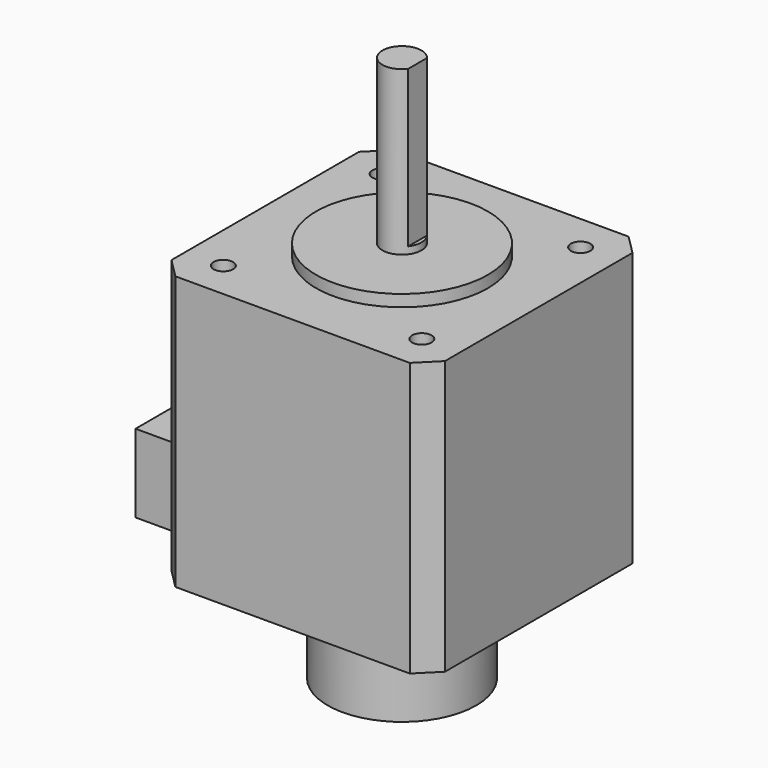
from build123d import *

# Parameters (mm, degrees)
F0_W      = 35
F0_H      = 35
F1_DEPTH  = 35
F2_SIZE   = 2.5
F3_R      = 11
F4_DEPTH  = 1.5
F5_R      = 2.5
F6_DEPTH  = 0.9
F7_W      = 16.5
F7_H      = 10
F8_DEPTH  = 10
F10_DEPTH = 20
F12_D     = 2.5
F12_DEPTH = 4.5
F12_TIP   = 0.7510757738
F20_R     = 9.5
F20_R_2   = 2.5
F21_DEPTH = 12.5
F22_DEPTH = 7.5


with BuildPart() as f1:
    # F0 (on Top) → F1 (new body)
    with BuildSketch(Plane.XY):
        Rectangle(F0_W, F0_H)
    extrude(amount=F1_DEPTH)

    # F2
    f2_edges = [f1.edges().sort_by_distance(p)[0] for p in [
        (17.5, -17.5, 17.5),
        (-17.5, -17.5, 17.5),
        (-17.5, 17.5, 17.5),
        (17.5, 17.5, 17.5),
    ]]
    chamfer(f2_edges, length=F2_SIZE)

    # F3 (on face) → F4 (join)
    with BuildSketch(Plane.XY.offset(35)):
        Circle(F3_R)
    extrude(amount=F4_DEPTH)

    # F5 (on face) → F6 (join)
    with BuildSketch(Plane.XY.offset(36.5)):
        Circle(F5_R)
    extrude(amount=F6_DEPTH)

    # F7 (on face) → F8 (join)
    with BuildSketch(Plane(origin=(-17.5, 0, 0), x_dir=(0, -1, 0), z_dir=(-1, 0, 0))):
        with Locations((0, 5)):
            Rectangle(F7_W, F7_H)
    extrude(amount=F8_DEPTH)

    # F9 (on face) → F10 (join)
    with BuildSketch(Plane.XY.offset(37.4)):
        with BuildLine():
            ThreePointArc((2, 1.5), (-2.5, 0), (2, -1.5))
            Line((2, -1.5), (2, 1.5))
        make_face()
    extrude(amount=F10_DEPTH)

    # F12
    with Locations(Plane.XY.offset(35)):
        with Locations((-12.7, 12.7), (12.7, 12.7), (12.7, -12.7), (-12.7, -12.7)):
            Hole(F12_D / 2, depth=F12_DEPTH)
            with Locations((0, 0, -(F12_DEPTH + F12_TIP / 2))):  # 118° drill point
                Cone(0, F12_D / 2, F12_TIP, mode=Mode.SUBTRACT)


with BuildPart() as f14:
    # F13 (on Front) → F14 (revolve)
    with BuildSketch(Plane.XZ):
        Polygon((8.9, 6.9), (8.9, 8), (2.5, 8), (2.5, -8), (8.9, -8), (8.9, -0.5), (6, -0.5), (6, 6.9), align=None)
    revolve(axis=Axis((0, 0, 0), (0, 0, 1)))


with BuildPart() as f16:
    # F15 (on Front) → F16 (revolve)
    with BuildSketch(Plane.XZ):
        Polygon((2.5, 4.25), (2.5, -4.25), (9, -4.25), (9, -3.25), (6, -3.25), (6, 3.25), (9, 3.25), (9, 4.25), align=None)
    revolve(axis=Axis((0, 0, 0), (0, 0, 1)))


with BuildPart() as f18:
    # F17 (on Front) → F18 (revolve)
    with BuildSketch(Plane.XZ):
        Polygon((-3, -9.5), (-3, 0), (-6, 0), (-6, -5.9), (-5.7, -5.9), (-5.7, -6.9), (-6, -6.9), (-6, -9.5), align=None)
    revolve(axis=Axis((0, 0, -4.75), (0, 0, 1)))

    # F19: F18 across plane


with BuildPart() as f18_1:
    add(f18.part)
    add(f18.part.mirror(Plane.XY))


with BuildPart() as f21:
    # F20 (on Top) → F21 (new body, symmetric)
    with BuildSketch(Plane.XY):
        Circle(F20_R)
        Circle(F20_R_2, mode=Mode.SUBTRACT)
    extrude(amount=F21_DEPTH, both=True)

    # F20 (on Top) → F22 (join, symmetric)
    with BuildSketch(Plane.XY):
        Circle(F20_R_2)
    extrude(amount=F22_DEPTH, both=True)


solid = Compound([f1.part, f14.part, f16.part, f18_1.part, f21.part])
